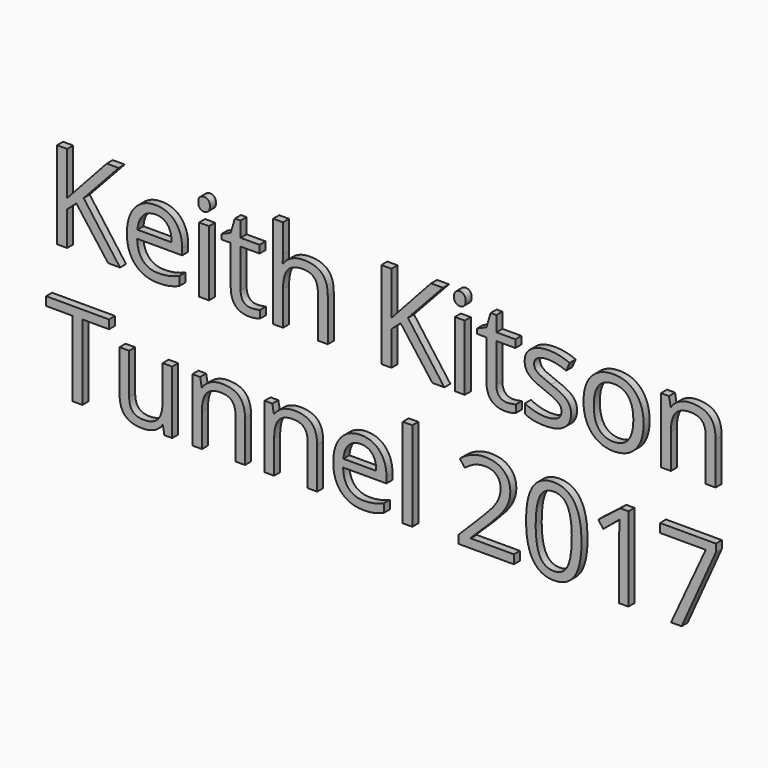
from build123d import *

# Parameters (mm, degrees)
F0_TEXT_SIZE   = 81.0331729552
F0_TEXT_SIZE_2 = 77.9980500487
F1_DEPTH       = 5


# Not quite as in the source:
# - Text() gives the source's letters only with a copy of the font that has no kerning and outlines rounded to 1/6400 em; it was checked with that copy


with BuildPart() as f1:
    # F0 (on Front) → F1 (new body)
    with BuildSketch(Plane.XZ):
        with Locations((0, 141.6561154723)):
            Text('Keith Kitson', F0_TEXT_SIZE, font='Open Sans', text_align=(TextAlign.LEFT, TextAlign.BOTTOM))
        with Locations((0, 53.3122309445)):
            Text('Tunnel 2017', F0_TEXT_SIZE_2, font='Open Sans', text_align=(TextAlign.LEFT, TextAlign.BOTTOM))
    extrude(amount=F1_DEPTH)


solid = f1.part
